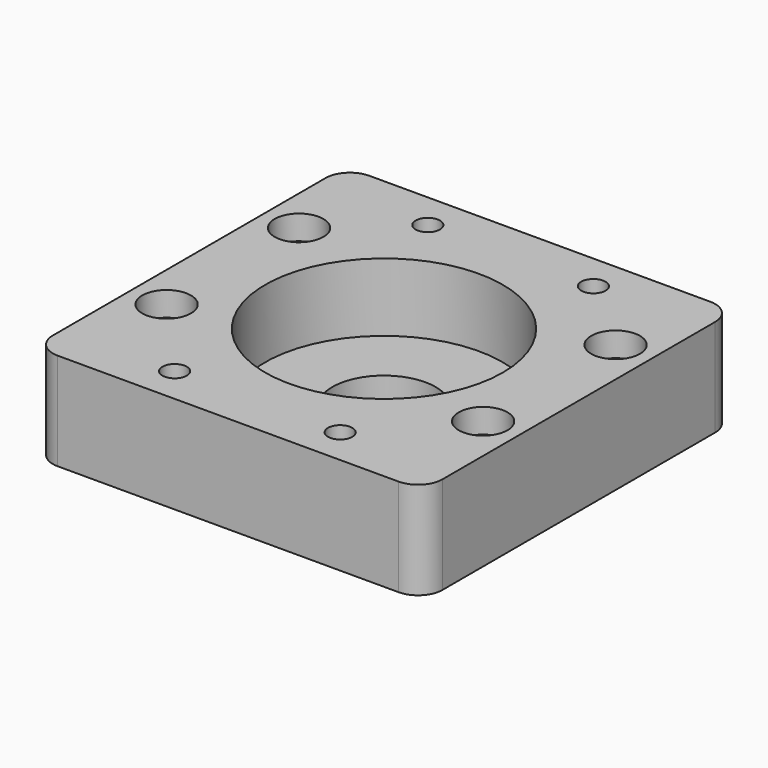
from build123d import *

# Parameters (mm, degrees)
F1_DEPTH        = 25.4
F2_R            = 13.49375
F3_DEPTH        = 25.4
F4_R            = 30.99943
F4_R_2          = 13.49375
F5_DEPTH        = 17.78
F6_R            = 31.0007
F6_R_2          = 12.50061
F7_DEPTH        = 16.99768
F8_DEPTH        = 16.99768
F11_D           = 6.35
F11_DEPTH       = 38.1
F11_CBORE_D     = 12.7
F11_CBORE_DEPTH = 6.35
F11_TIP         = 1.9077324654
F13_D           = 6.35
F13_DEPTH       = 38.1
F13_CBORE_D     = 12.7
F13_CBORE_DEPTH = 6.35
F13_TIP         = 1.9077324654


# Not quite as in the source:
# - a feature names something its author has since deleted; it is built from what else it names


with BuildPart() as f1:
    # F0 (on Top) → F1 (new body)
    with BuildSketch(Plane.XY):
        with BuildLine():
            ThreePointArc((-50.8, -44.45), (-48.9401280605, -48.9401280605), (-44.45, -50.8))
            Line((-44.45, -50.8), (-31.75, -50.8))
            Line((-31.75, -50.8), (31.75, -50.8))
            Line((31.75, -50.8), (44.45, -50.8))
            ThreePointArc((44.45, -50.8), (48.9401280605, -48.9401280605), (50.8, -44.45))
            Line((50.8, -44.45), (50.8, 44.45))
            ThreePointArc((50.8, 44.45), (48.9401280605, 48.9401280605), (44.45, 50.8))
            Line((44.45, 50.8), (-44.45, 50.8))
            ThreePointArc((-44.45, 50.8), (-48.9401280605, 48.9401280605), (-50.8, 44.45))
            Line((-50.8, 44.45), (-50.8, -44.45))
        make_face()
    extrude(amount=F1_DEPTH)

    # F2 (on face) → F3 (cut)
    with BuildSketch(Plane.XY.offset(25.4)):
        Circle(F2_R)
    extrude(amount=-F3_DEPTH, mode=Mode.SUBTRACT)

    # F4 (on face) → F5 (cut)
    with BuildSketch(Plane.XY.offset(25.4)):
        Circle(F4_R)
        Circle(F4_R_2, mode=Mode.SUBTRACT)
    extrude(amount=-F5_DEPTH, mode=Mode.SUBTRACT)

    # F11
    with Locations(Plane(origin=(0, 0, 0), x_dir=(1, 0, 0), z_dir=(0, 0, -1))):
        with Locations((-21.59, -41.275), (21.59, -41.275), (-21.59, 41.275), (21.59, 41.275)):
            CounterBoreHole(F11_D / 2, F11_CBORE_D / 2, F11_CBORE_DEPTH, depth=F11_DEPTH)
            with Locations((0, 0, -(F11_DEPTH + F11_TIP / 2))):  # 118° drill point
                Cone(0, F11_D / 2, F11_TIP, mode=Mode.SUBTRACT)

    # F13
    with Locations(Plane.XY.offset(25.4)):
        with Locations((-41.275, 23.8990909091), (-41.275, -19.2809090909), (41.275, 23.8990909091), (41.275, -19.2809090909)):
            CounterBoreHole(F13_D / 2, F13_CBORE_D / 2, F13_CBORE_DEPTH, depth=F13_DEPTH)
            with Locations((0, 0, -(F13_DEPTH + F13_TIP / 2))):  # 118° drill point
                Cone(0, F13_D / 2, F13_TIP, mode=Mode.SUBTRACT)


with BuildPart() as f7:
    # F6 (on Top) → F7 (new body)
    with BuildSketch(Plane.XY):
        with Locations((-113.8032615222, 0)):
            Circle(F6_R)
        with Locations((-113.8032615222, 0)):
            Circle(F6_R_2, mode=Mode.SUBTRACT)
    extrude(amount=F7_DEPTH)


with BuildPart() as f8:
    # F6 (on Top) → F8 (new body)
    with BuildSketch(Plane.XY):
        with Locations((-113.8032615222, 0)):
            Circle(F6_R)
        with Locations((-113.8032615222, 0)):
            Circle(F6_R_2, mode=Mode.SUBTRACT)
    extrude(amount=F8_DEPTH)


solid = f1.part
